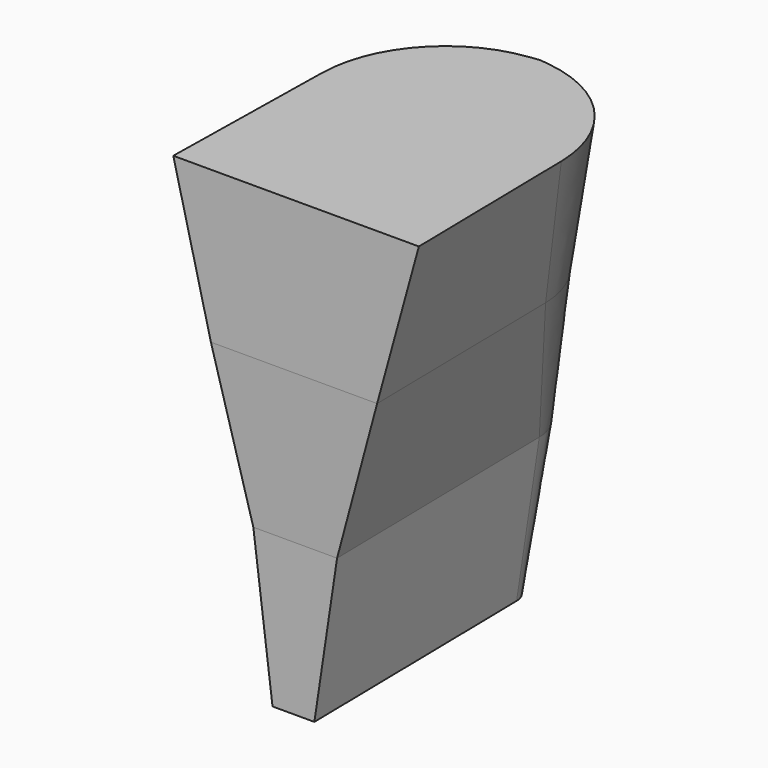
from build123d import *


# Not quite as in the source:
# - ends of sketch curves that miss each other by under 0.0002 mm in the source are joined


with BuildPart() as f7:
    # F3 (on offset) → F7 section 0
    with BuildSketch(Plane.XY.offset(304.8)):
        with BuildLine():
            Line((-124.6491538, -192.8961344), (124.6491538, -192.8961344))
            Line((124.6491538, -192.8961344), (121.4234808, -8.0974946))
            ThreePointArc((121.4234808, -8.0974946), (88.9728976434, 74.4979752801), (10.3676203953, 115.6836712928))
            Line((10.3676203953, 115.6836712928), (0, 116.9940256))
            Line((0, 116.9940256), (-10.3676196, 115.683665))
            ThreePointArc((-10.3676196, 115.683665), (-88.9728976434, 74.4979752801), (-121.4234675032, -8.0974948321))
            Line((-121.4234675032, -8.0974948321), (-124.6491538, -192.8961344))
        make_face()
    # F4 (on offset) → F7 section 1
    with BuildSketch(Plane.XY.offset(152.4)):
        with BuildLine():
            Line((-84.3707736, -195.5275744), (84.3707736, -195.5275744))
            Line((84.3707736, -195.5275744), (80.5558968, 23.025862))
            ThreePointArc((80.5558968, 23.025862), (58.8138267519, 81.0794433275), (5.3479189082, 112.4535200809))
            Line((5.3479189082, 112.4535200809), (0, 113.4807484))
            Line((0, 113.4807484), (-5.3479192, 112.4535216))
            ThreePointArc((-5.3479192, 112.4535216), (-58.8138267519, 81.0794433275), (-80.5558986997, 23.0258620332))
            Line((-80.5558986997, 23.0258620332), (-84.3707736, -195.5275744))
        make_face()
    loft()


with BuildPart() as f8:
    # F4 (on offset) → F8 section 0
    with BuildSketch(Plane.XY.offset(152.4)):
        with BuildLine():
            Line((-84.3707736, -195.5275744), (84.3707736, -195.5275744))
            Line((84.3707736, -195.5275744), (80.5558968, 23.025862))
            ThreePointArc((80.5558968, 23.025862), (58.8138267519, 81.0794433275), (5.3479189082, 112.4535200809))
            Line((5.3479189082, 112.4535200809), (0, 113.4807484))
            Line((0, 113.4807484), (-5.3479192, 112.4535216))
            ThreePointArc((-5.3479192, 112.4535216), (-58.8138267519, 81.0794433275), (-80.5558986997, 23.0258620332))
            Line((-80.5558986997, 23.0258620332), (-84.3707736, -195.5275744))
        make_face()
    # F5 (on Top) → F8 section 1
    with BuildSketch(Plane.XY):
        with BuildLine():
            Line((0, 112.5638084), (-0.83693, 112.4030518))
            ThreePointArc((-0.83693, 112.4030518), (-27.2036803488, 96.9309041513), (-37.9258027274, 68.3017429289))
            Line((-37.9258027274, 68.3017429289), (-42.50436, -194.0035744))
            Line((-42.50436, -194.0035744), (42.50436, -194.0035744))
            Line((42.50436, -194.0035744), (37.9258068, 68.301743))
            ThreePointArc((37.9258068, 68.301743), (27.2036803488, 96.9309041513), (0.8369291121, 112.4030471776))
            Line((0.8369291121, 112.4030471776), (0, 112.5638084))
        make_face()
    loft()


with BuildPart() as f9:
    # F5 (on Top) → F9 section 0
    with BuildSketch(Plane.XY):
        with BuildLine():
            Line((0, 112.5638084), (-0.83693, 112.4030518))
            ThreePointArc((-0.83693, 112.4030518), (-27.2036803488, 96.9309041513), (-37.9258027274, 68.3017429289))
            Line((-37.9258027274, 68.3017429289), (-42.50436, -194.0035744))
            Line((-42.50436, -194.0035744), (42.50436, -194.0035744))
            Line((42.50436, -194.0035744), (37.9258068, 68.301743))
            ThreePointArc((37.9258068, 68.301743), (27.2036803488, 96.9309041513), (0.8369291121, 112.4030471776))
            Line((0.8369291121, 112.4030471776), (0, 112.5638084))
        make_face()
    # F6 (on offset) → F9 section 1
    with BuildSketch(Plane.XY.offset(-152.4)):
        with BuildLine():
            Line((-16.7496236, 66.163063), (-21.3281768, -196.1422544))
            Line((-21.3281768, -196.1422544), (21.1761832, -196.1422544))
            Line((21.1761832, -196.1422544), (16.59763, 66.163063))
            ThreePointArc((16.59763, 66.163063), (11.8850820526, 78.7459853527), (0.2965144503, 85.5462079895))
            Line((0.2965144503, 85.5462079895), (-0.0618236, 85.6184216))
            Line((-0.0618236, 85.6184216), (-0.443738, 85.5461332))
            ThreePointArc((-0.443738, 85.5461332), (-12.0328808906, 78.7452835073), (-16.7496236, 66.163063))
        make_face()
    loft()


solid = Compound([f7.part, f8.part, f9.part])
